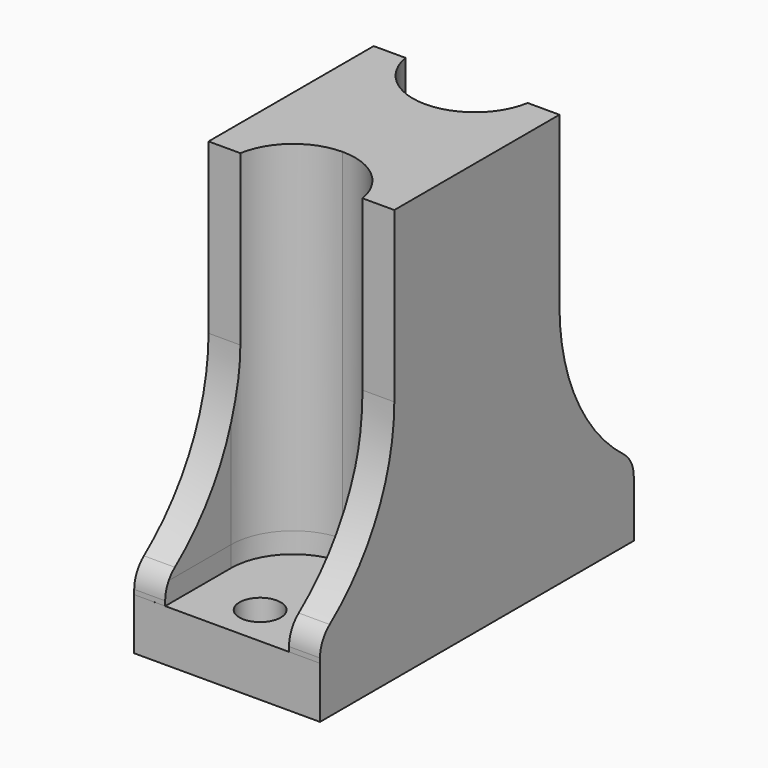
from build123d import *

# Parameters (mm, degrees)
F0_W         = 22.86
F0_H         = 48.26
F1_DEPTH     = 50.8
F2_W         = 15.24
F2_H         = 6.35
F3_DEPTH     = 41.91
F4_T1_DEPTH  = 3.81
F4_T3_DEPTH  = 3.81
F4_T8_DEPTH  = 56.8427535009
F4_T14_DEPTH = 56.8427535009
F4_T20_DEPTH = 56.8427535009
F4_T26_DEPTH = 56.8427535009
F5_R         = 7.61999
F6_DEPTH     = 2.54
F7_R         = 3.81
F8_R         = 2.54
F9_DEPTH     = 25.4


# Not quite as in the source:
# - a fillet or chamfer that OpenCascade refuses, or shapes differently, is made with other operations: its cross-section is extruded or revolved along the edge and cut away or added
# - a fillet or chamfer is up to 0.001 mm smaller than in the source, because OpenCascade refuses the exact size


with BuildPart() as f1:
    # F0 (on Top) → F1 (new body)
    with BuildSketch(Plane.XY):
        Rectangle(F0_W, F0_H)
    extrude(amount=F1_DEPTH)

    # F2 (on face) → F3 (cut)
    with BuildSketch(Plane.XY.offset(50.8)):
        Polygon((11.43, 24.13), (-11.43, 24.13), (-11.43, 12.7), (-7.62, 12.7), (7.62, 12.7), (11.43, 12.7), align=None)
        with Locations((0, 9.525)):
            Rectangle(F2_W, F2_H)
        Polygon((-11.43, -12.7), (-11.43, -24.13), (11.43, -24.13), (11.43, -12.7), (7.62, -12.7), (-7.62, -12.7), align=None)
        with Locations((0, -9.525)):
            Rectangle(F2_W, F2_H)
    extrude(amount=-F3_DEPTH, mode=Mode.SUBTRACT)

    # F4: fillet of radius 25.4 on 4 edges, made by hand

    # F4_s2 → F4_t1 (join)
    with BuildSketch(Plane.YZ.offset(-11.43)):
        with BuildLine():
            ThreePointArc((-24.1299175004, 8.889874725), (-15.7392117545, 18.0547879388), (-12.69985, 30.1031013998))
            Line((-12.69985, 30.1031013998), (-12.19185, 30.1031013998))
            ThreePointArc((-12.19185, 30.1031013998), (-12.192, 19.4965506999), (-12.192, 8.89))
            Line((-12.192, 8.89), (-12.7, 8.382))
            ThreePointArc((-12.7, 8.382), (-18.4149587502, 8.382), (-23.8505188504, 8.4656101915))
            Line((-23.8505188504, 8.4656101915), (-24.1299175004, 8.889874725))
        make_face()
        with BuildLine():
            ThreePointArc((24.1299175004, 8.889874725), (15.7392117545, 18.0547879388), (12.69985, 30.1031013998))
            Line((12.69985, 30.1031013998), (12.19185, 30.1031013998))
            ThreePointArc((12.19185, 30.1031013998), (12.192, 19.4965506999), (12.192, 8.89))
            Line((12.192, 8.89), (12.7, 8.382))
            ThreePointArc((12.7, 8.382), (18.4149587502, 8.382), (23.8505188504, 8.4656101915))
            Line((23.8505188504, 8.4656101915), (24.1299175004, 8.889874725))
        make_face()
    extrude(amount=F4_T1_DEPTH)

    # F4_s4 → F4_t3 (join)
    with BuildSketch(Plane.YZ.offset(7.62)):
        with BuildLine():
            ThreePointArc((-24.1299175004, 8.889874725), (-15.7392117545, 18.0547879388), (-12.69985, 30.1031013998))
            Line((-12.69985, 30.1031013998), (-12.19185, 30.1031013998))
            ThreePointArc((-12.19185, 30.1031013998), (-12.192, 19.4965506999), (-12.192, 8.89))
            Line((-12.192, 8.89), (-12.7, 8.382))
            ThreePointArc((-12.7, 8.382), (-18.4149587502, 8.382), (-23.8505188504, 8.4656101915))
            Line((-23.8505188504, 8.4656101915), (-24.1299175004, 8.889874725))
        make_face()
        with BuildLine():
            ThreePointArc((24.1299175004, 8.889874725), (15.7392117545, 18.0547879388), (12.69985, 30.1031013998))
            Line((12.69985, 30.1031013998), (12.19185, 30.1031013998))
            ThreePointArc((12.19185, 30.1031013998), (12.192, 19.4965506999), (12.192, 8.89))
            Line((12.192, 8.89), (12.7, 8.382))
            ThreePointArc((12.7, 8.382), (18.4149587502, 8.382), (23.8505188504, 8.4656101915))
            Line((23.8505188504, 8.4656101915), (24.1299175004, 8.889874725))
        make_face()
    extrude(amount=F4_T3_DEPTH)


with BuildPart() as f4_tool6:
    # F4_s7 → F4_t8 (new body)
    with BuildSketch(Plane.YZ.offset(45.4127535009)):
        with BuildLine():
            ThreePointArc((-24.1299175004, 8.889874725), (-15.7392117545, 18.0547879388), (-12.69985, 30.1031013998))
            Line((-12.69985, 30.1031013998), (-12.19185, 30.1031013998))
            ThreePointArc((-12.19185, 30.1031013998), (-12.192, 19.4965506999), (-12.192, 8.89))
            Line((-12.192, 8.89), (-12.7, 8.382))
            ThreePointArc((-12.7, 8.382), (-18.4149587502, 8.382), (-23.8505188504, 8.4656101915))
            Line((-23.8505188504, 8.4656101915), (-24.1299175004, 8.889874725))
        make_face()
    extrude(amount=-F4_T8_DEPTH)

    split(bisect_by=Plane.YZ.offset(11.43), keep=Keep.BOTTOM)

    split(bisect_by=Plane.YZ.offset(7.62), keep=Keep.TOP)


with BuildPart() as f1_1:
    add(f1.part)

    # F4_t5: union F4_tool6
    add(f4_tool6.part)


with BuildPart() as f4_tool12:
    # F4_s13 → F4_t14 (new body)
    with BuildSketch(Plane.YZ.offset(11.43)):
        with BuildLine():
            ThreePointArc((-24.1299175004, 8.889874725), (-15.7392117545, 18.0547879388), (-12.69985, 30.1031013998))
            Line((-12.69985, 30.1031013998), (-12.19185, 30.1031013998))
            ThreePointArc((-12.19185, 30.1031013998), (-12.192, 19.4965506999), (-12.192, 8.89))
            Line((-12.192, 8.89), (-12.7, 8.382))
            ThreePointArc((-12.7, 8.382), (-18.4149587502, 8.382), (-23.8505188504, 8.4656101915))
            Line((-23.8505188504, 8.4656101915), (-24.1299175004, 8.889874725))
        make_face()
    extrude(amount=-F4_T14_DEPTH)

    split(bisect_by=Plane.YZ.offset(-11.43), keep=Keep.TOP)

    split(bisect_by=Plane.YZ.offset(-7.62), keep=Keep.BOTTOM)


with BuildPart() as f1_2:
    add(f1_1.part)

    # F4_t11: union F4_tool12
    add(f4_tool12.part)


with BuildPart() as f4_tool18:
    # F4_s19 → F4_t20 (new body)
    with BuildSketch(Plane.YZ.offset(-11.43)):
        with BuildLine():
            ThreePointArc((24.1299175004, 8.889874725), (15.7392117545, 18.0547879388), (12.69985, 30.1031013998))
            Line((12.69985, 30.1031013998), (12.19185, 30.1031013998))
            ThreePointArc((12.19185, 30.1031013998), (12.192, 19.4965506999), (12.192, 8.89))
            Line((12.192, 8.89), (12.7, 8.382))
            ThreePointArc((12.7, 8.382), (18.4149587502, 8.382), (23.8505188504, 8.4656101915))
            Line((23.8505188504, 8.4656101915), (24.1299175004, 8.889874725))
        make_face()
    extrude(amount=F4_T20_DEPTH)

    split(bisect_by=Plane.YZ.offset(11.43), keep=Keep.BOTTOM)

    split(bisect_by=Plane.YZ.offset(7.62), keep=Keep.TOP)


with BuildPart() as f1_3:
    add(f1_2.part)

    # F4_t17: union F4_tool18
    add(f4_tool18.part)


with BuildPart() as f4_tool24:
    # F4_s25 → F4_t26 (new body)
    with BuildSketch(Plane.YZ.offset(-45.4127535009)):
        with BuildLine():
            ThreePointArc((24.1299175004, 8.889874725), (15.7392117545, 18.0547879388), (12.69985, 30.1031013998))
            Line((12.69985, 30.1031013998), (12.19185, 30.1031013998))
            ThreePointArc((12.19185, 30.1031013998), (12.192, 19.4965506999), (12.192, 8.89))
            Line((12.192, 8.89), (12.7, 8.382))
            ThreePointArc((12.7, 8.382), (18.4149587502, 8.382), (23.8505188504, 8.4656101915))
            Line((23.8505188504, 8.4656101915), (24.1299175004, 8.889874725))
        make_face()
    extrude(amount=F4_T26_DEPTH)

    split(bisect_by=Plane.YZ.offset(-11.43), keep=Keep.TOP)

    split(bisect_by=Plane.YZ.offset(-7.62), keep=Keep.BOTTOM)


with BuildPart() as f1_4:
    add(f1_3.part)

    # F4_t23: union F4_tool24
    add(f4_tool24.part)

    # F5 (radius 7.62 in the source; OpenCascade refuses exactly that, so slightly less here)
    f5_edges = [f1_4.edges().sort_by_distance(p)[0] for p in [
        (7.62, 6.35, 29.845),
        (-7.62, 6.35, 29.845),
        (7.62, -6.35, 29.845),
        (-7.62, -6.35, 29.845),
    ]]
    fillet(f5_edges, radius=F5_R)

    # F6 (cut): faces of the model
    f6_faces = [f1_4.faces().sort_by_distance(p)[0] for p in [
        (0, 15.9681179393, 8.89),
        (0, -15.9681179393, 8.89),
    ]]
    extrude(f6_faces, amount=-F6_DEPTH, mode=Mode.SUBTRACT)

    # F7
    f7_edges = [f1_4.edges().sort_by_distance(p)[0] for p in [
        (9.525, 24.129727, 8.89),
        (9.525, -24.129727, 8.89),
        (-9.525, 24.129727, 8.89),
        (-9.525, -24.129727, 8.89),
    ]]
    fillet(f7_edges, radius=F7_R)

    # F8 (on face) → F9 (cut)
    with BuildSketch(Plane.XY.offset(6.35)):
        with Locations((0, -19.05)):
            Circle(F8_R)
        with Locations((0, 19.05)):
            Circle(F8_R)
    extrude(amount=-F9_DEPTH, mode=Mode.SUBTRACT)


solid = f1_4.part
